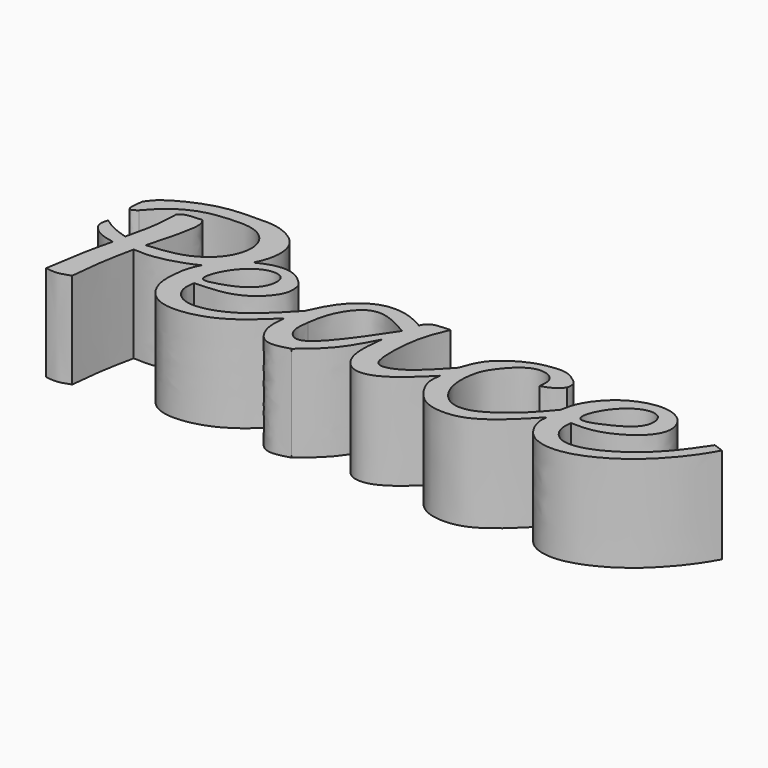
from build123d import *

# Parameters (mm, degrees)
F1_DEPTH = 15
F3_DEPTH = 8


with BuildPart() as f1:
    # F0 (on Top) → F1 (new body)
    with BuildSketch(Plane.XY):
        with BuildLine():
            add(Edge.make_bspline(
                [(-29.5197498053, 16.0896964371), (-29.2959248841, 17.0866768453), (-28.9570431175, 17.9865364975), (-28.5339232006, 18.7932092998)],
                knots=[0, 0, 0, 0, 0.1193114698, 0.1193114698, 0.1193114698, 0.1193114698], degree=3))
            add(Edge.make_bspline(
                [(-29.5197498053, 16.0896964371), (-29.7031065197, 14.6563172426), (-30.080045439, 11.7096217462), (-28.1322871252, 8.759925381), (-26.4865215868, 8.0765383318)],
                knots=[0, 0, 0, 0, 0.2073575456, 0.4262790671, 0.4262790671, 0.4262790671, 0.4262790671], degree=3))
            add(Edge.make_bspline(
                [(-26.4865215868, 8.0765383318), (-24.3712413413, 7.1981901762), (-17.8840994319, 8.2079095342), (-13.895871726, 12.139582434), (-11.8636386469, 14.1429975629)],
                knots=[0.4262790671, 0.4262790671, 0.4262790671, 0.4262790671, 0.7076559455, 1, 1, 1, 1], degree=3))
            add(Edge.make_bspline(
                [(-11.8636386469, 14.1429975629), (-11.9919670944, 13.0883304188), (-12.2526083771, 10.9462504463), (-10.2153785321, 7.2023382975), (-7.5198727613, 7.9751970563), (-6.1371922493, 8.3716409281)],
                knots=[0, 0, 0, 0, 0.3208255575, 0.6516122221, 1, 1, 1, 1], degree=3))
            add(Edge.make_bspline(
                [(-6.1371922493, 8.3716409281), (-4.7049770612, 9.5508191577), (-1.8004106416, 11.944123887), (0.0085061179, 15.4262155687), (0.9252529708, 17.1948950738)],
                knots=[0, 0, 0, 0, 0.4928718937, 1, 1, 1, 1], degree=3))
            add(Edge.make_bspline(
                [(0.9252529708, 17.1948950738), (0.7002885074, 15.2129187205), (0.2948956357, 11.6686773245), (2.8534995196, 8.3256503296), (7.2214848398, 9.0430540833), (10.5903189017, 12.2451424426), (12.4796722084, 14.1429975629)],
                knots=[0, 0, 0, 0, 0.2662560325, 0.4748550688, 0.6918347611, 1, 1, 1, 1], degree=3))
            add(Edge.make_bspline(
                [(12.4796722084, 14.1429975629), (12.3567270292, 13.3382773369), (12.14040693, 11.6866274324), (14.1680771363, 8.3563764669), (16.6960843798, 6.843858018), (20.9356335968, 6.7199377707), (25.0508891214, 9.0723771082), (28.001238583, 12.0543664551), (29.5260921121, 13.7017956004)],
                knots=[0, 0, 0, 0, 0.1309459503, 0.2919621729, 0.4354540719, 0.6027228467, 0.784505056, 1, 1, 1, 1], degree=3))
            add(Edge.make_bspline(
                [(29.5260921121, 13.7017956004), (29.4494344459, 13.1510419203), (29.3115775332, 11.9578711835), (31.001212058, 8.2394328011), (36.1145843581, 7.0708416903), (42.2117822652, 9.6169760573), (46.573863691, 13.1346350854), (49.9266045093, 17.0857546913), (51.1581874034, 19.2222665215), (51.7203956842, 20.1976578683)],
                knots=[0, 0, 0, 0, 0.0899502167, 0.2212376244, 0.3723173697, 0.5483148575, 0.7139379788, 0.8700324828, 1, 1, 1, 1], degree=3))
            Line((51.7203956842, 20.1976578683), (50.1595586538, 20.7686945796))
            add(Edge.make_bspline(
                [(32.7983126044, 14.3592404202), (32.7153503568, 13.7323555449), (32.5362242327, 12.3788307643), (34.177987249, 9.747083146), (38.8427355373, 9.7604999377), (45.8804799663, 14.4091846262), (48.7479970496, 18.6708504577), (50.1595586538, 20.7686945796)],
                knots=[0, 0, 0, 0, 0.130090907, 0.2808829393, 0.4700062965, 0.7391057348, 1, 1, 1, 1], degree=3))
            add(Edge.make_bspline(
                [(29.588283971, 16.3035858423), (29.7616917917, 17.2053776187), (30.1627716399, 19.291157298), (33.5068853144, 23.2810073199), (38.1596043126, 24.8599408195), (41.2541002931, 24.2873570254), (43.0490114044, 22.683768941), (43.7218716906, 20.0178969278), (41.6710895913, 16.88834866), (36.7785570041, 14.2784160551), (34.0517720177, 14.3337871939), (32.7983126044, 14.3592404202)],
                knots=[0, 0, 0, 0, 0.1000330229, 0.231369205, 0.3598860143, 0.4603773571, 0.5477091259, 0.6387126974, 0.7479317597, 0.8841282645, 1, 1, 1, 1], degree=3))
            add(Edge.make_bspline(
                [(23.645831272, 19.6124818176), (23.7203833838, 20.2123241708), (23.8704148875, 21.3933142156), (22.6701217375, 22.8924812944), (19.5221839217, 23.1427632594), (16.3109184961, 19.4772592399), (15.2895614031, 17.2986171252), (14.8792866219, 13.0982142101), (17.05717861, 9.3483199148), (21.2088747712, 8.5887501402), (26.7442270709, 12.8463793621), (28.7028105399, 15.2281055095), (29.588283971, 16.3035858423)],
                knots=[0, 0, 0, 0, 0.0707743039, 0.1396140029, 0.228929762, 0.3440556474, 0.4292761333, 0.536753367, 0.6438866817, 0.7459339665, 0.8852224949, 1, 1, 1, 1], degree=3))
            add(Edge.make_bspline(
                [(26.526927948, 21.3411394507), (26.1385483593, 20.9400395262), (25.3505362754, 20.126218212), (24.2194502874, 19.7853498294), (23.645831272, 19.6124818176)],
                knots=[0, 0, 0, 0, 0.4928599404, 1, 1, 1, 1], degree=3))
            add(Edge.make_bspline(
                [(12.8943044692, 17.1948950738), (13.3425896626, 18.491787842), (14.2804655004, 21.2142228005), (18.8593458781, 23.903692294), (21.393850445, 24.4249510687), (24.0737893185, 24.6930231444), (25.7581339132, 23.4584551751), (26.7110830768, 22.704102983), (26.5899543358, 21.8076092017), (26.526927948, 21.3411394507)],
                knots=[0, 0, 0, 0, 0.1840283222, 0.3856193225, 0.5329945244, 0.6763715981, 0.8040129767, 0.8980060108, 1, 1, 1, 1], degree=3))
            add(Edge.make_bspline(
                [(5.9051825665, 24.39795807), (5.2796526411, 22.9712299099), (3.9353644531, 19.9050894014), (3.7075616843, 12.9009672388), (4.9490431647, 11.3184163953), (8.496299722, 12.3856851943), (11.2468870531, 15.3909715866), (12.8943044692, 17.1948950738)],
                knots=[0, 0, 0, 0, 0.2170119072, 0.4664184993, 0.5823552154, 0.7497429619, 1, 1, 1, 1], degree=3))
            add(Edge.make_bspline(
                [(2.1475991234, 22.9039788246), (2.3428401586, 23.3003573055), (2.8310561944, 24.2915338294), (4.7522735677, 24.358045116), (5.9051825665, 24.39795807)],
                knots=[0, 0, 0, 0, 0.3999070512, 1, 1, 1, 1], degree=3))
            add(Edge.make_bspline(
                [(-11.1623937264, 17.1948950738), (-10.5398511892, 18.5628349484), (-9.2707374001, 21.3594980591), (-5.248213519, 24.7374533554), (-0.7298831893, 24.4906309653), (1.2322453903, 23.4086829672), (2.1475991234, 22.9039788246)],
                knots=[0, 0, 0, 0, 0.2603156398, 0.5312425545, 0.7812722516, 1, 1, 1, 1], degree=3))
            add(Edge.make_bspline(
                [(-26.3120550662, 14.4988177344), (-26.4222931202, 13.7768911895), (-26.6615542892, 12.2101495597), (-24.3282508745, 9.2469865739), (-17.4297661724, 10.5963680293), (-13.3925098593, 14.8444387075), (-11.1623937264, 17.1948950738)],
                knots=[0, 0, 0, 0, 0.1694155161, 0.367717612, 0.6506295652, 1, 1, 1, 1], degree=3))
            add(Edge.make_bspline(
                [(-15.95112037, 21.9937769871), (-15.7966520892, 21.216655299), (-15.4154688091, 19.2989425314), (-19.5008131736, 14.743263195), (-23.9492657643, 14.5836147697), (-26.3120550662, 14.4988177344)],
                knots=[0, 0, 0, 0, 0.2421048194, 0.5974450468, 1, 1, 1, 1], degree=3))
            add(Edge.make_bspline(
                [(-24.0700956622, 23.2628666258), (-23.2776920759, 23.6864516212), (-20.1311153039, 24.8738854789), (-17.7451969535, 24.2725213112), (-15.95112037, 21.9937769871)],
                knots=[0.4293270672, 0.4293270672, 0.4293270672, 0.4293270672, 0.5741513965, 1, 1, 1, 1], degree=3))
            add(Edge.make_bspline(
                [(-28.5339232006, 18.7932092998), (-27.4805344869, 19.3586454328), (-25.8445145474, 20.5733086864), (-24.5247192992, 22.4099469585), (-24.0700956622, 23.2628666258)],
                knots=[0.2164607486, 0.2164607486, 0.2164607486, 0.2164607486, 0.2921979477, 0.349944774, 0.349944774, 0.349944774, 0.349944774], degree=3))
        make_face()
        with BuildLine():
            add(Edge.make_bspline(
                [(-26.1831432581, 16.0770304501), (-26.5705475824, 16.5915824541), (-25.5236781222, 19.8500439887), (-22.3942558617, 22.7980811841), (-19.5909944076, 22.9806135847), (-18.455931748, 21.7897345319), (-18.7610605958, 19.3004890899), (-20.8794412927, 17.1979951748), (-24.0654910281, 16.0934411171), (-25.8961329296, 15.6958221609), (-26.1831432581, 16.0770304501)],
                knots=[0, 0, 0, 0, 0.1402941833, 0.3022737646, 0.4209424648, 0.5087922195, 0.6222593339, 0.7517086902, 0.8960623898, 1, 1, 1, 1], degree=3))
        make_face(mode=Mode.SUBTRACT)
        with BuildLine():
            add(Edge.make_bspline(
                [(-8.9235752821, 15.0464298204), (-9.0646859983, 14.0808295866), (-9.3271993781, 12.2844884749), (-7.5404688212, 10.3547407663), (-5.0207003169, 11.4635558948), (-1.2953094882, 16.3396092098), (0.5618805634, 19.1479797333), (1.4483764535, 20.4885043204)],
                knots=[0, 0, 0, 0, 0.1779548177, 0.3310557971, 0.4918670148, 0.7574519621, 1, 1, 1, 1], degree=3))
            add(Edge.make_bspline(
                [(-8.9235752821, 15.0464298204), (-8.7718449134, 16.1215699221), (-8.449567237, 18.4051843159), (-5.958882275, 22.3564152791), (-2.6113827935, 22.7845317726), (-0.0046509708, 21.3102749358), (1.4483764535, 20.4885043204)],
                knots=[0, 0, 0, 0, 0.2372477596, 0.5039179524, 0.7234771856, 1, 1, 1, 1], degree=3))
        make_face(mode=Mode.SUBTRACT)
        with BuildLine():
            add(Edge.make_bspline(
                [(32.9581163824, 15.9508809447), (32.4202349789, 16.4558861758), (33.5372547907, 19.9580854994), (37.2715590249, 23.1501136882), (40.5087156051, 22.7034723084), (40.7973008496, 19.1294802461), (37.0761086127, 16.8016116704), (33.520287852, 15.4230702953), (32.9581163824, 15.9508809447)],
                knots=[0, 0, 0, 0, 0.1648006178, 0.3622570844, 0.4996763079, 0.6407463677, 0.8277571879, 1, 1, 1, 1], degree=3))
        make_face(mode=Mode.SUBTRACT)
        with BuildLine():
            add(Edge.make_bspline(
                [(-37.63435781, 16.8396867812), (-36.792774095, 16.780997693), (-34.7988064496, 16.6419460296), (-30.9505530887, 17.6314034567), (-28.9442923194, 18.5729320891), (-28.5339232006, 18.7932092998)],
                knots=[0, 0, 0, 0, 0.0785934067, 0.1869557735, 0.2164607486, 0.2164607486, 0.2164607486, 0.2164607486], degree=3))
            add(Edge.make_bspline(
                [(-28.5339232006, 18.7932092998), (-27.4345002025, 20.8892454247), (-25.7663401568, 22.3561270188), (-24.0700956622, 23.2628666258)],
                knots=[0.1193114698, 0.1193114698, 0.1193114698, 0.1193114698, 0.4293270672, 0.4293270672, 0.4293270672, 0.4293270672], degree=3))
            add(Edge.make_bspline(
                [(-24.0700956622, 23.2628666258), (-23.6593076141, 24.0335463196), (-22.7421148215, 26.4102337749), (-23.137984421, 30.4038791076), (-27.4676487416, 32.7905284602), (-31.2729050018, 32.6073591163), (-36.826013927, 32.6764343172), (-43.5764893816, 29.296188472), (-44.3511297111, 27.8653610127), (-44.7214916348, 27.40371041)],
                knots=[0.349944774, 0.349944774, 0.349944774, 0.349944774, 0.4021235525, 0.501487602, 0.6002895059, 0.6916758101, 0.8050336314, 0.932529676, 1, 1, 1, 1], degree=3))
            add(Edge.make_bspline(
                [(-44.7214916348, 27.40371041), (-44.8994629954, 26.0626483288), (-45.0946801171, 24.4835341745), (-44.1135664101, 24.9118394746), (-43.5886271298, 25.354931131)],
                knots=[0, 0, 0, 0, 0.5888424904, 1, 1, 1, 1], degree=3))
            add(Edge.make_bspline(
                [(-43.5886271298, 25.354931131), (-42.8698733446, 26.1771232695), (-41.3516522159, 27.9138368734), (-37.6044812798, 30.0075770022), (-33.4805276823, 30.4938502102), (-29.1108568661, 30.5796693033), (-26.2024184332, 27.6396314104), (-26.8391241832, 22.8646700552), (-31.1110959696, 19.1945600689), (-35.1137430617, 18.8342796295), (-37.1904708445, 18.6473522335)],
                knots=[0, 0, 0, 0, 0.1099985997, 0.2323496608, 0.3556770614, 0.4783969704, 0.5912201693, 0.7150692357, 0.8521669233, 1, 1, 1, 1], degree=3))
            add(Edge.make_bspline(
                [(-37.1904708445, 18.6473522335), (-36.2452841246, 22.0915778581), (-34.9373760502, 26.85754675), (-35.7489373077, 27.8983428661), (-35.9740070999, 28.1869862229)],
                knots=[0, 0, 0, 0, 0.7226706054, 1, 1, 1, 1], degree=3))
            add(Edge.make_bspline(
                [(-35.9740070999, 28.1869862229), (-36.9473854974, 28.1461458568), (-38.5225068768, 28.0800579573), (-39.1300566376, 27.578966837), (-39.3621586263, 27.3875351995)],
                knots=[0, 0, 0, 0, 0.6179704055, 1, 1, 1, 1], degree=3))
            add(Edge.make_bspline(
                [(-40.5884683132, 18.8792515546), (-40.2150467083, 20.4148384075), (-39.4958540428, 23.3723073574), (-39.4055666832, 26.0838761589), (-39.3621586263, 27.3875351995)],
                knots=[0, 0, 0, 0, 0.519223322, 1, 1, 1, 1], degree=3))
            add(Edge.make_bspline(
                [(-44.8954962194, 20.8873717549), (-44.2531018535, 20.4531410381), (-42.9511384226, 19.5730702534), (-41.3829206703, 19.1125494232), (-40.5884683132, 18.8792515546)],
                knots=[0, 0, 0, 0, 0.4934043082, 1, 1, 1, 1], degree=3))
            add(Edge.make_bspline(
                [(-40.9114956856, 16.8396867812), (-41.8524511704, 17.0332486566), (-43.6302677156, 17.3989593732), (-45.3793010236, 19.2701406063), (-45.0464709781, 20.3827031771), (-44.8954962194, 20.8873717549)],
                knots=[0, 0, 0, 0, 0.3805574121, 0.7190151655, 1, 1, 1, 1], degree=3))
            add(Edge.make_bspline(
                [(-42.9034940898, 6.2811863609), (-42.5282867495, 8.7092642449), (-41.8715441541, 12.9592401912), (-41.1995633303, 15.6753381611), (-40.9114956856, 16.8396867812)],
                knots=[0, 0, 0, 0, 0.5713156768, 1, 1, 1, 1], degree=3))
            add(Edge.make_bspline(
                [(-39.1709432006, 6.7238314077), (-39.8278750159, 6.4831096726), (-41.0996635916, 6.0170839064), (-42.3156266432, 6.1951155046), (-42.9034940898, 6.2811863609)],
                knots=[0, 0, 0, 0, 0.5165416862, 1, 1, 1, 1], degree=3))
            add(Edge.make_bspline(
                [(-39.1709432006, 6.7238314077), (-39.0103435648, 8.4121673837), (-38.6882375031, 11.7983721501), (-37.986309728, 15.1560976908), (-37.63435781, 16.8396867812)],
                knots=[0, 0, 0, 0, 0.4985924043, 1, 1, 1, 1], degree=3))
        make_face()
        with BuildLine():
            add(Edge.make_bspline(
                [(-28.5339232006, 18.7932092998), (-27.4345002025, 20.8892454247), (-25.7663401568, 22.3561270188), (-24.0700956622, 23.2628666258)],
                knots=[0.1193114698, 0.1193114698, 0.1193114698, 0.1193114698, 0.4293270672, 0.4293270672, 0.4293270672, 0.4293270672], degree=3))
            add(Edge.make_bspline(
                [(-28.5339232006, 18.7932092998), (-27.4805344869, 19.3586454328), (-25.8445145474, 20.5733086864), (-24.5247192992, 22.4099469585), (-24.0700956622, 23.2628666258)],
                knots=[0.2164607486, 0.2164607486, 0.2164607486, 0.2164607486, 0.2921979477, 0.349944774, 0.349944774, 0.349944774, 0.349944774], degree=3))
        make_face()
    extrude(amount=F1_DEPTH)

    # F2 (on face) → F3 (cut)
    with BuildSketch(Plane(origin=(0, 0, 0), x_dir=(1, 0, 0), z_dir=(0, 0, -1))):
        with BuildLine():
            add(Edge.make_bspline(
                [(-10.8508163852, -16.8396867812), (-10.7296307855, -17.2534176083), (-10.0615694827, -19.0006588286), (-8.3529720443, -20.9384151347), (-7.0483875461, -22.4179718643)],
                knots=[0.7108527882, 0.7108527882, 0.7108527882, 0.7108527882, 0.7792241978, 1, 1, 1, 1], degree=3))
            add(Edge.make_bspline(
                [(-7.0483875461, -22.4179718643), (-6.3163591305, -22.8738471409), (-4.8069631438, -23.8138329369), (-1.7302002729, -23.9716679693), (0.8010059378, -22.8550193078), (2.192996908, -22.2409386188)],
                knots=[0, 0, 0, 0, 0.2976632276, 0.6137626239, 1, 1, 1, 1], degree=3))
            add(Edge.make_bspline(
                [(2.192996908, -22.2409386188), (2.4880592632, -22.821458311), (3.0509290652, -23.9288750939), (4.8706024236, -23.5806795), (4.9023641291, -23.586692247), (4.9055325799, -23.5872920603)],
                knots=[0, 0, 0, 0, 0.4979570054, 0.9499177243, 1, 1, 1, 1], degree=3))
            add(Edge.make_bspline(
                [(4.9055325799, -23.5872920603), (4.4510058057, -22.3116314774), (3.4909011294, -19.6170318177), (3.0391181383, -14.7910435875), (3.1805692887, -10.0730016245), (8.1697383697, -11.3513396748), (11.1586247418, -14.3489503875), (12.8943044692, -16.0896964371)],
                knots=[0, 0, 0, 0, 0.1894426737, 0.4001629987, 0.5757515496, 0.7536341824, 1, 1, 1, 1], degree=3))
            add(Edge.make_bspline(
                [(12.8943044692, -16.0896964371), (13.3780422907, -17.6002957945), (14.398563108, -20.7871421031), (19.4290474001, -24.0733124717), (24.3757872517, -24.6374487783), (25.4396750089, -22.7295136647), (25.909839198, -21.8863394111)],
                knots=[0, 0, 0, 0, 0.2611253493, 0.5508848865, 0.8015224428, 1, 1, 1, 1], degree=3))
            add(Edge.make_bspline(
                [(24.3736859411, -20.4363279045), (24.8359211893, -20.5167710988), (25.7296026643, -20.6722992479), (25.8511562708, -21.4910619998), (25.909839198, -21.8863394111)],
                knots=[0, 0, 0, 0, 0.5172259481, 1, 1, 1, 1], degree=3))
            add(Edge.make_bspline(
                [(20.0718734413, -23.1036730111), (20.5630551283, -23.2508018814), (21.6197803429, -23.5673340143), (24.0350893656, -22.9178291887), (24.2591664756, -21.2756163714), (24.3736859411, -20.4363279045)],
                knots=[0, 0, 0, 0, 0.2980684864, 0.6412626806, 1, 1, 1, 1], degree=3))
            add(Edge.make_bspline(
                [(16.3197554648, -9.8780253902), (15.7009075463, -10.5841415242), (14.252803598, -12.2364530711), (14.3824353524, -17.8422120473), (17.2374237424, -21.76739179), (19.1999535971, -22.6926125803), (20.0718734413, -23.1036730111)],
                knots=[0, 0, 0, 0, 0.2166283577, 0.5069102937, 0.7809283263, 1, 1, 1, 1], degree=3))
            add(Edge.make_bspline(
                [(16.3197554648, -9.8780253902), (16.8583557359, -9.3195191307), (18.079709566, -8.0530255997), (22.5184672186, -8.4446116974), (26.8740422184, -12.699491466), (29.588283971, -15.3509834781)],
                knots=[0, 0, 0, 0, 0.2291515783, 0.5196342685, 1, 1, 1, 1], degree=3))
            add(Edge.make_bspline(
                [(29.588283971, -15.3509834781), (29.9621376985, -16.7523676873), (30.7592926907, -19.7404893404), (34.9845504029, -23.8896061696), (39.9204465773, -24.4656263591), (41.358829702, -23.3956400749), (41.9589616358, -22.9492131621)],
                knots=[0, 0, 0, 0, 0.2584122072, 0.5510031487, 0.8126664975, 1, 1, 1, 1], degree=3))
            add(Edge.make_bspline(
                [(41.9589616358, -22.9492131621), (42.4319765157, -22.1369673047), (43.4575029697, -20.3759664368), (40.9423804788, -17.1121736029), (36.316584547, -14.8248195554), (33.7064524272, -14.8429941384), (32.5055792928, -14.8513559252)],
                knots=[0, 0, 0, 0, 0.2102028564, 0.4557332107, 0.7495929956, 1, 1, 1, 1], degree=3))
            add(Edge.make_bspline(
                [(32.5055792928, -14.8513559252), (32.2655755615, -14.1418231509), (31.746961418, -12.6086231041), (33.1881977361, -9.209313012), (38.2702334212, -8.8185511693), (43.8102592876, -12.251939226), (48.2540719109, -17.1427092706), (49.6770269424, -19.2255186927), (50.2742230892, -20.0996473432)],
                knots=[0, 0, 0, 0, 0.1222348254, 0.2641321821, 0.4336403042, 0.6412575458, 0.8494403501, 1, 1, 1, 1], degree=3))
            add(Edge.make_bspline(
                [(50.8655682206, -19.6877475828), (50.8402367992, -19.8440569998), (50.7884076057, -20.1638728871), (50.4481701331, -20.1213746476), (50.2742230892, -20.0996473432)],
                knots=[0, 0, 0, 0, 0.4887481306, 1, 1, 1, 1], degree=3))
            add(Edge.make_bspline(
                [(30.0516951829, -13.7017956004), (30.011923763, -13.3135162084), (29.9180746027, -12.397288047), (30.8309772214, -10.1363092733), (32.7113889345, -8.2438905135), (37.742354595, -7.6462563593), (44.6613789322, -11.5251907056), (48.6918851197, -16.8279360717), (50.8655682206, -19.6877475828)],
                knots=[0, 0, 0, 0, 0.0907050864, 0.2140380259, 0.3424859786, 0.5151562921, 0.7385200455, 1, 1, 1, 1], degree=3))
            add(Edge.make_bspline(
                [(29.5260921121, -14.1429975629), (29.7308336423, -14.1830027763), (30.1290613695, -14.2608139814), (30.0769933694, -13.8845905899), (30.0516951829, -13.7017956004)],
                knots=[0, 0, 0, 0, 0.51413178, 1, 1, 1, 1], degree=3))
            add(Edge.make_bspline(
                [(13.039524667, -15.0368940085), (12.9680735442, -14.2640690119), (12.8071627541, -12.5236361693), (14.2377269186, -8.626234007), (17.9803303313, -6.8577884135), (23.0456873037, -7.9491436179), (27.1440891752, -11.8663221508), (29.5260921121, -14.1429975629)],
                knots=[0, 0, 0, 0, 0.1475878158, 0.3323736717, 0.513356351, 0.7171613137, 1, 1, 1, 1], degree=3))
            add(Edge.make_bspline(
                [(0.8712882991, -18.0178601295), (1.1628098019, -18.0989470212), (2.0826760713, -18.3548084101), (0.6972937953, -14.5205818123), (1.6125484963, -10.4330139197), (4.7915508812, -9.1329263544), (8.3292962357, -10.5884252185), (11.3132824924, -13.4065836001), (13.039524667, -15.0368940085)],
                knots=[0, 0, 0, 0, 0.0775536263, 0.2447125312, 0.4331527413, 0.5886121137, 0.7620112634, 1, 1, 1, 1], degree=3))
            add(Edge.make_bspline(
                [(-6.0108904727, -9.1779595241), (-5.233984304, -9.7757841348), (-3.574743134, -11.0525602069), (-1.0586546904, -14.1036026486), (0.2150356567, -16.6868665048), (0.8712882991, -18.0178601295)],
                knots=[0, 0, 0, 0, 0.2991502037, 0.6388961164, 1, 1, 1, 1], degree=3))
            add(Edge.make_bspline(
                [(-6.0108904727, -9.1779595241), (-6.7801168866, -8.8534439838), (-8.1977155156, -8.2553979772), (-10.1426321245, -8.5397482889), (-11.6088393518, -11.348898855), (-11.3762302206, -13.767824688), (-11.2208807841, -14.9300452322)],
                knots=[0, 0, 0, 0, 0.1456249331, 0.2683705366, 0.4277572637, 0.6079840904, 0.6079840904, 0.6079840904, 0.6079840904], degree=3))
            add(Edge.make_bspline(
                [(-11.2208807841, -14.9300452322), (-11.1322114415, -15.5934099274), (-11.0331470541, -16.2172050783), (-10.8508163852, -16.8396867812)],
                knots=[0.6079840904, 0.6079840904, 0.6079840904, 0.6079840904, 0.7108527882, 0.7108527882, 0.7108527882, 0.7108527882], degree=3))
        make_face()
        with BuildLine():
            add(Edge.make_bspline(
                [(-26.7109647393, -15.0057654828), (-26.8175097727, -14.5248273583), (-27.0585710973, -13.4366904672), (-27.1874111849, -10.5043356266), (-24.4644145349, -9.3548648369), (-21.6845792811, -9.1847854769), (-17.1947967776, -10.7223116068), (-13.200121395, -14.574298294), (-10.8508163852, -16.8396867812)],
                knots=[0, 0, 0, 0, 0.1135035299, 0.2568051312, 0.3988538946, 0.545513168, 0.7327121508, 1, 1, 1, 1], degree=3))
            add(Edge.make_bspline(
                [(-11.2208807841, -14.9300452322), (-11.1322114415, -15.5934099274), (-11.0331470541, -16.2172050783), (-10.8508163852, -16.8396867812)],
                knots=[0.6079840904, 0.6079840904, 0.6079840904, 0.6079840904, 0.7108527882, 0.7108527882, 0.7108527882, 0.7108527882], degree=3))
            add(Edge.make_bspline(
                [(-21.7123329639, -8.3952061832), (-20.9278646945, -8.5494622208), (-19.0928417675, -8.9102969119), (-15.2694146643, -11.5933808791), (-12.6068012138, -13.7878166055), (-11.2208807841, -14.9300452322)],
                knots=[0, 0, 0, 0, 0.2636462484, 0.6167195401, 1, 1, 1, 1], degree=3))
            add(Edge.make_bspline(
                [(-28.0247703195, -19.5612795651), (-28.0059820438, -19.3290457561), (-27.9567336684, -18.7203077305), (-28.5728511311, -16.7169794088), (-29.6142404306, -13.2972442393), (-27.847328568, -9.395796282), (-24.8305324411, -8.025543159), (-22.7529568311, -8.2718400648), (-21.7123329639, -8.3952061832)],
                knots=[0, 0, 0, 0, 0.0905121599, 0.2372531103, 0.4324401689, 0.6378507132, 0.8186053064, 1, 1, 1, 1], degree=3))
            add(Edge.make_bspline(
                [(-38.3674576879, -16.8396867812), (-38.2719279582, -17.0086059817), (-38.0250344695, -17.4451721783), (-36.4055092729, -17.1435225639), (-32.5017154358, -17.3882725477), (-29.5831241347, -18.8048901772), (-28.0247703195, -19.5612795651)],
                knots=[0, 0, 0, 0, 0.1214193624, 0.3138044052, 0.6336124476, 1, 1, 1, 1], degree=3))
            add(Edge.make_bspline(
                [(-39.9188883603, -7.1144397371), (-39.7552580084, -8.5084019598), (-39.4071797805, -11.4736702913), (-38.7275799998, -14.9810917991), (-38.3674576879, -16.8396867812)],
                knots=[0, 0, 0, 0, 0.470096486, 1, 1, 1, 1], degree=3))
            add(Edge.make_bspline(
                [(-42.1402566135, -7.1144397371), (-41.8353414333, -6.9623413619), (-41.1822556863, -6.6365678765), (-40.3582037602, -6.9482675849), (-39.9188883603, -7.1144397371)],
                knots=[0, 0, 0, 0, 0.4668838382, 1, 1, 1, 1], degree=3))
            add(Edge.make_bspline(
                [(-40.5497029424, -17.2587186098), (-40.5276848889, -16.9620620306), (-40.4587611511, -16.0334295211), (-41.3906717487, -10.9402193492), (-41.8994776496, -8.3433429529), (-42.1402566135, -7.1144397371)],
                knots=[0, 0, 0, 0, 0.1982520215, 0.6205939295, 1, 1, 1, 1], degree=3))
            add(Edge.make_bspline(
                [(-44.5638298988, -20.0012885034), (-44.6850938639, -19.8999340439), (-44.9763405631, -19.6565051593), (-44.4623458106, -18.5087504487), (-42.1432861578, -17.7678450045), (-40.5497029424, -17.2587186098)],
                knots=[0, 0, 0, 0, 0.1824530229, 0.4382080086, 1, 1, 1, 1], degree=3))
            add(Edge.make_bspline(
                [(-38.7404747307, -27.40371041), (-38.8743185194, -26.5127681159), (-39.1832659987, -24.4562335647), (-39.0915886054, -18.3335658139), (-41.3525904463, -18.3085270063), (-43.9916547136, -19.874594638), (-44.4338187552, -19.9725007916), (-44.5638298988, -20.0012885034)],
                knots=[0, 0, 0, 0, 0.227253207, 0.5245615516, 0.684581247, 0.9072562467, 1, 1, 1, 1], degree=3))
            add(Edge.make_bspline(
                [(-36.5948267281, -27.40371041), (-36.9672874094, -27.5249271039), (-37.7007850985, -27.7636426767), (-38.3975286049, -27.5224356263), (-38.7404747307, -27.40371041)],
                knots=[0, 0, 0, 0, 0.507787123, 1, 1, 1, 1], degree=3))
            add(Edge.make_bspline(
                [(-37.582103163, -19.3632859737), (-37.3230599101, -20.1682293417), (-36.7700975068, -21.886488413), (-36.4524480935, -25.3330653181), (-36.551611107, -26.7752157349), (-36.5948267281, -27.40371041)],
                knots=[0, 0, 0, 0, 0.3321087353, 0.7089304288, 1, 1, 1, 1], degree=3))
            add(Edge.make_bspline(
                [(-44.3913675845, -25.4102554172), (-43.8276001413, -25.9061959029), (-42.6161255277, -26.9719177987), (-40.4460955014, -29.3081878284), (-36.5369072489, -30.5258843062), (-31.7687749912, -31.2249177549), (-27.7817348141, -30.3614019195), (-25.7832784184, -28.2038540798), (-26.2259194867, -23.8692712904), (-27.7347873479, -20.3335708226), (-34.1035071341, -18.2897630619), (-38.081539379, -17.7759051298), (-37.7173375523, -18.9334643626), (-37.582103163, -19.3632859737)],
                knots=[0, 0, 0, 0, 0.0747278296, 0.1605819378, 0.2589762129, 0.3675478156, 0.4641698645, 0.5426074975, 0.6410392291, 0.7343960625, 0.8620018932, 0.9487589344, 1, 1, 1, 1], degree=3))
            add(Edge.make_bspline(
                [(-44.3913675845, -25.4102554172), (-44.4302329117, -25.8174389825), (-44.5105305765, -26.6587001195), (-43.9160676998, -28.0645756825), (-40.2217484958, -30.6086919232), (-35.1551338819, -32.0774654701), (-29.7069616128, -32.3099314769), (-26.165739226, -31.3167998082), (-23.713786481, -28.9334836974), (-23.9461947641, -25.714689298), (-24.521709684, -24.1718003997), (-24.794459343, -23.4405901283)],
                knots=[0, 0, 0, 0, 0.0686757196, 0.1418873915, 0.2712381293, 0.4188286542, 0.5645460048, 0.6835861137, 0.7935834, 0.902174461, 1, 1, 1, 1], degree=3))
            add(Edge.make_bspline(
                [(-24.794459343, -23.4405901283), (-25.0333263631, -22.9774845064), (-25.517412188, -22.038958682), (-24.5257615579, -22.4808695759), (-24.0234304219, -22.7047242224)],
                knots=[0, 0, 0, 0, 0.4934394023, 1, 1, 1, 1], degree=3))
            add(Edge.make_bspline(
                [(-24.0234304219, -22.7047242224), (-23.5578701031, -22.9628500708), (-22.5871772017, -23.5010422633), (-20.7437044254, -24.181523205), (-18.7271931196, -23.8382919364), (-17.2118872687, -22.7833397685), (-16.072604669, -21.3094646039), (-16.6205649891, -18.92745817), (-18.5307479878, -16.754417514), (-22.4433835718, -14.871054175), (-25.2842759886, -14.9607303446), (-26.7109647393, -15.0057654828)],
                knots=[0, 0, 0, 0, 0.0913395188, 0.1904428255, 0.2906419517, 0.3870501292, 0.4801206855, 0.5856129228, 0.7060992647, 0.8524038184, 1, 1, 1, 1], degree=3))
        make_face()
    extrude(amount=-F3_DEPTH, mode=Mode.SUBTRACT)


solid = f1.part
